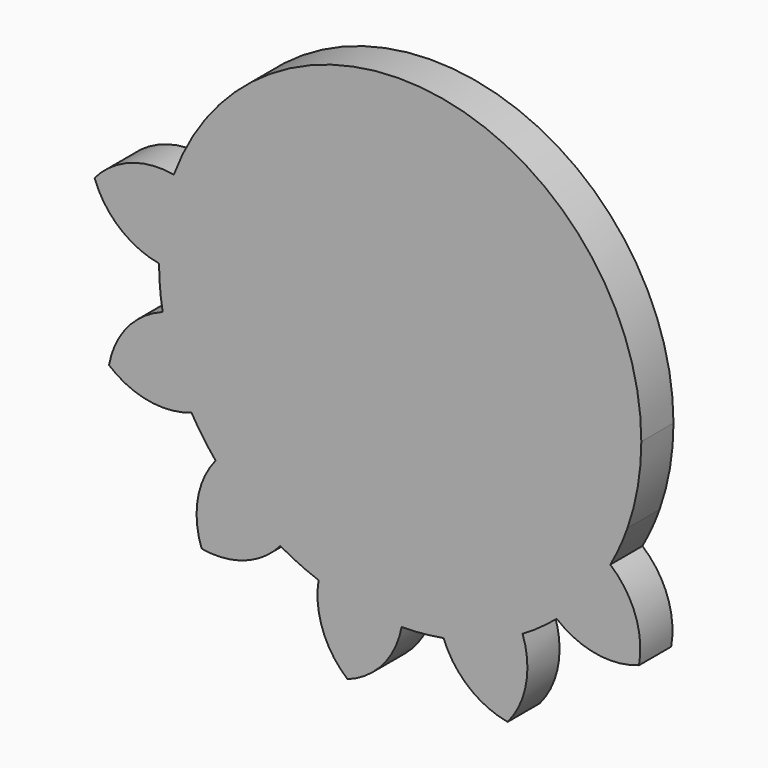
from build123d import *

# Parameters (mm, degrees)
F1_DEPTH = 3.175


# Not quite as in the source:
# - a feature names something its author has since deleted; it is built from what else it names


with BuildPart() as f1:
    # F0 (on Front) → F1 (new body)
    with BuildSketch(Plane.XZ):
        with BuildLine():
            ThreePointArc((-19.05, 0), (-18.7565324084, 3.330914591), (-17.8851714423, 6.5592028846))
            ThreePointArc((-17.8851714423, 6.5592028846), (-21.3208303202, 6.2628506055), (-24.1480220477, 4.2883725643))
            ThreePointArc((-24.1480220477, 4.2883725643), (-22.1735440066, 1.4611808368), (-19.05, 0))
        make_face()
        with BuildLine():
            ThreePointArc((17.9570302857, -6.3598398815), (18.774769332, -3.2265363052), (19.05, 0))
            ThreePointArc((19.05, 0), (3.330914591, 18.7565324084), (-17.8851714423, 6.5592028846))
            ThreePointArc((-17.8851714423, 6.5592028846), (-18.7565324084, 3.330914591), (-19.05, 0))
            ThreePointArc((-19.05, 0), (-18.9787164623, -1.6464572402), (-18.7653993235, -3.2805926645))
            ThreePointArc((-18.7653993235, -3.2805926645), (-17.902768373, -6.5110202414), (-16.4886138833, -9.5408653804))
            ThreePointArc((-16.4886138833, -9.5408653804), (-15.5953963885, -10.940114784), (-14.5837536932, -12.2562893331))
            ThreePointArc((-14.5837536932, -12.2562893331), (-12.2164908848, -14.6171081429), (-9.4729601013, -16.5277199552))
            ThreePointArc((-9.4729601013, -16.5277199552), (-7.9923386115, -17.2923400244), (-6.4505607615, -17.9246413036))
            ThreePointArc((-6.4505607615, -17.9246413036), (-3.2177031841, -18.7762852082), (0.114253165, -19.0496573779))
            ThreePointArc((0.114253165, -19.0496573779), (1.7773096461, -18.9669098807), (3.4267873399, -18.7392536812))
            ThreePointArc((3.4267873399, -18.7392536812), (6.6502136181, -17.8515309941), (9.6687925813, -16.4139254909))
            ThreePointArc((9.6687925813, -16.4139254909), (11.058239811, -15.5118610193), (12.3640641678, -14.4924952045))
            ThreePointArc((12.3640641678, -14.4924952045), (14.707623832, -12.107365577), (16.5980379903, -9.3492050396))
            ThreePointArc((16.5980379903, -9.3492050396), (17.3420662524, -7.8838593403), (17.9570302857, -6.3598398815))
        make_face()
        with BuildLine():
            ThreePointArc((-16.4886138833, -9.5408653804), (-17.902768373, -6.5110202414), (-18.7653993235, -3.2805926645))
            ThreePointArc((-18.7653993235, -3.2805926645), (-21.5590287963, -5.2571672852), (-23.0027619685, -8.3598834163))
            ThreePointArc((-23.0027619685, -8.3598834163), (-19.9027732819, -9.816837479), (-16.4886138833, -9.5408653804))
        make_face()
        with BuildLine():
            ThreePointArc((-9.4729601013, -16.5277199552), (-12.2164908848, -14.6171081429), (-14.5837536932, -12.2562893331))
            ThreePointArc((-14.5837536932, -12.2562893331), (-15.9914516234, -15.352990661), (-15.6868096556, -18.7409643694))
            ThreePointArc((-15.6868096556, -18.7409643694), (-12.286729337, -18.4573983143), (-9.4729601013, -16.5277199552))
        make_face()
        with BuildLine():
            ThreePointArc((-4.1604686233, -24.0732680372), (-1.3577089131, -22.1276679749), (0.114253165, -19.0496573779))
            ThreePointArc((0.114253165, -19.0496573779), (-3.2177031841, -18.7762852082), (-6.4505607615, -17.9246413036))
            ThreePointArc((-6.4505607615, -17.9246413036), (-6.1149672512, -21.3004400299), (-4.1604686233, -24.0732680372))
        make_face()
        with BuildLine():
            ThreePointArc((8.4877873574, -22.928007958), (9.9447352105, -19.8280535223), (9.6687925813, -16.4139254909))
            ThreePointArc((9.6687925813, -16.4139254909), (6.6502136181, -17.8515309941), (3.4267873399, -18.7392536812))
            ThreePointArc((3.4267873399, -18.7392536812), (5.4050438072, -21.50087086), (8.4877873574, -22.928007958))
        make_face()
        with BuildLine():
            ThreePointArc((18.8688683105, -15.6120556451), (18.5725160314, -12.1763967671), (16.5980379903, -9.3492050396))
            ThreePointArc((16.5980379903, -9.3492050396), (14.707623832, -12.107365577), (12.3640641678, -14.4924952045))
            ThreePointArc((12.3640641678, -14.4924952045), (15.4680658678, -15.9145025235), (18.8688683105, -15.6120556451))
        make_face()
    extrude(amount=F1_DEPTH)


solid = f1.part
